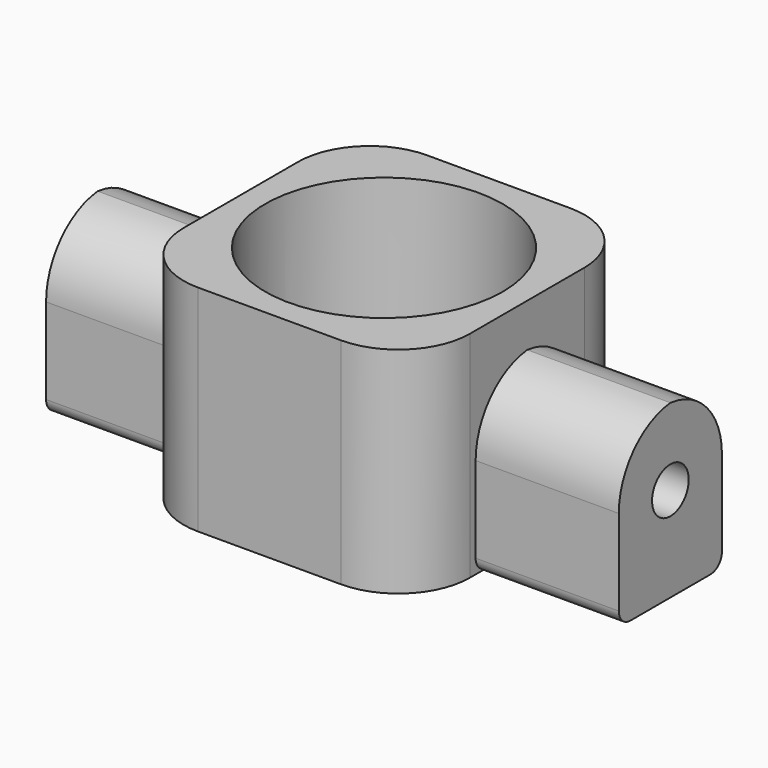
from build123d import *

# Parameters (mm, degrees)
F0_W        = 20
F0_H        = 20
F0_R        = 8.3
F1_DEPTH    = 15
F2_W        = 9
F2_H        = 12
F3_DEPTH    = 10
F4_W        = 9
F4_H        = 12
F4_R        = 1.6
F5_DEPTH    = 10
F6_DEPTH    = 30.001
F7_DEPTH    = 1.2
F8_T1_DEPTH = 40
F8_T3_DEPTH = 22.5
F8_T5_DEPTH = 22.5
F9_R        = 1


# Not quite as in the source:
# - a fillet or chamfer that OpenCascade refuses, or shapes differently, is made with other operations: its cross-section is extruded or revolved along the edge and cut away or added


with BuildPart() as f1:
    # F0 (on Top) → F1 (new body)
    with BuildSketch(Plane.XY):
        Rectangle(F0_W, F0_H)
        Circle(F0_R, mode=Mode.SUBTRACT)
    extrude(amount=F1_DEPTH)

    # F2 (on face) → F3 (join)
    with BuildSketch(Plane(origin=(-10, 0, 0), x_dir=(0, -1, 0), z_dir=(-1, 0, 0))):
        with Locations((0, 6)):
            Rectangle(F2_W, F2_H)
    extrude(amount=F3_DEPTH)

    # F4 (on face) → F5 (join)
    with BuildSketch(Plane.YZ.offset(10)):
        with Locations((0, 6)):
            Rectangle(F4_W, F4_H)
        with Locations((0, 6.6)):
            Circle(F4_R, mode=Mode.SUBTRACT)
    extrude(amount=F5_DEPTH)

    # F4 (on face) → F6 (cut, through all)
    with BuildSketch(Plane.YZ.offset(10)):
        with Locations((0, 6.6)):
            Circle(F4_R)
    extrude(amount=-F6_DEPTH, mode=Mode.SUBTRACT)

    # F0 (on Top) → F7 (join)
    with BuildSketch(Plane.XY):
        Circle(F0_R)
    extrude(amount=F7_DEPTH)

    # F8: fillet of radius 5 on 8 edges, made by hand

    # F8_s2 → F8_t1 (cut)
    with BuildSketch(Plane.XY.offset(-12.5)):
        with BuildLine():
            ThreePointArc((-10, -5), (-8.5355339059, -8.5355339059), (-5, -10))
            Line((-5, -10), (-10, -10))
            Line((-10, -10), (-10, -5))
        make_face()
        with BuildLine():
            ThreePointArc((10, -5), (8.5355339059, -8.5355339059), (5, -10))
            Line((5, -10), (10, -10))
            Line((10, -10), (10, -5))
        make_face()
        with BuildLine():
            ThreePointArc((-5, 10), (-8.5355339059, 8.5355339059), (-10, 5))
            Line((-10, 5), (-10, 10))
            Line((-10, 10), (-5, 10))
        make_face()
        with BuildLine():
            ThreePointArc((5, 10), (8.5355339059, 8.5355339059), (10, 5))
            Line((10, 5), (10, 10))
            Line((10, 10), (5, 10))
        make_face()
    extrude(amount=F8_T1_DEPTH, mode=Mode.SUBTRACT)

    # F8_s4 → F8_t3 (cut)
    with BuildSketch(Plane.YZ.offset(-32.5)):
        with BuildLine():
            ThreePointArc((4.5, 7), (3.0355339059, 10.5355339059), (-0.5, 12))
            Line((-0.5, 12), (4.5, 12))
            Line((4.5, 12), (4.5, 7))
        make_face()
        with BuildLine():
            ThreePointArc((0.5, 12), (-3.0355339059, 10.5355339059), (-4.5, 7))
            Line((-4.5, 7), (-4.5, 12))
            Line((-4.5, 12), (0.5, 12))
        make_face()
    extrude(amount=F8_T3_DEPTH, mode=Mode.SUBTRACT)

    # F8_s6 → F8_t5 (cut)
    with BuildSketch(Plane.YZ.offset(10)):
        with BuildLine():
            ThreePointArc((-0.5, 12), (3.0355339059, 10.5355339059), (4.5, 7))
            Line((4.5, 7), (4.5, 12))
            Line((4.5, 12), (-0.5, 12))
        make_face()
        with BuildLine():
            ThreePointArc((-4.5, 7), (-3.0355339059, 10.5355339059), (0.5, 12))
            Line((0.5, 12), (-4.5, 12))
            Line((-4.5, 12), (-4.5, 7))
        make_face()
    extrude(amount=F8_T5_DEPTH, mode=Mode.SUBTRACT)

    # F9
    f9_edges = [f1.edges().sort_by_distance(p)[0] for p in [
        (15, -4.5, 0),
        (15, 4.5, 0),
        (-15, 4.5, 0),
        (-15, -4.5, 0),
    ]]
    fillet(f9_edges, radius=F9_R)


solid = f1.part
